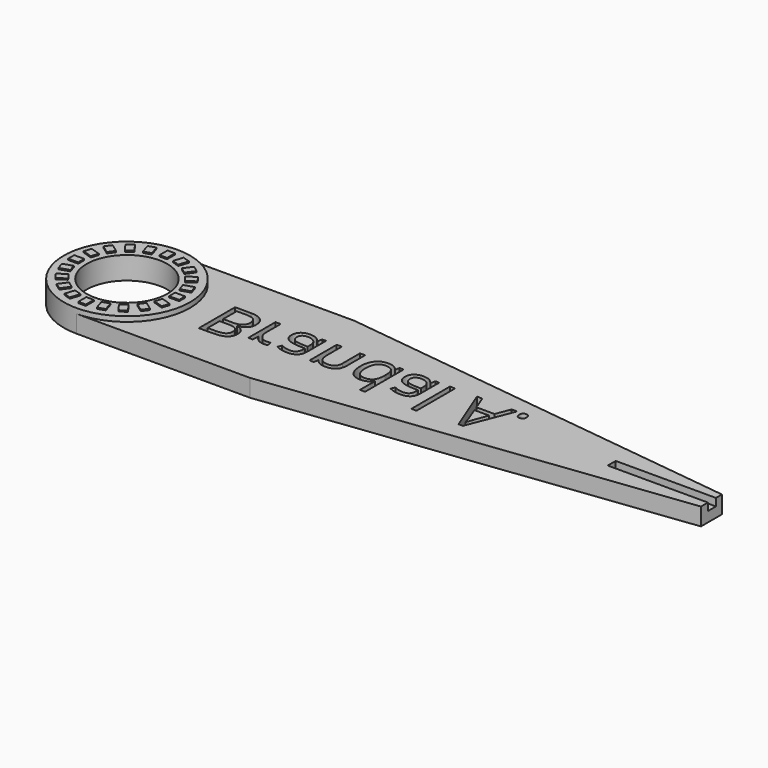
from build123d import *

# Parameters (mm, degrees)
F0_R         = 8.0699934722
F1_DEPTH     = 3.5
F2_R         = 12.6093648002
F2_R_2       = 8.0699934722
F3_DEPTH     = 1
F4_W         = 1.5
F4_H         = 2
F4_W_2       = 2
F4_H_2       = 1.5
F5_DEPTH     = 0.25
F6_W         = 20
F6_H         = 2
F7_DEPTH     = 1.5
F9_TEXT_SIZE = 12.6782884311
F10_DEPTH    = 4.751


# Not quite as in the source:
# - Text() gives the source's letters only with a copy of the font that has no kerning and outlines rounded to 1/6400 em; it was checked with that copy


with BuildPart() as f1:
    # F0 (on Top) → F1 (new body)
    with BuildSketch(Plane.XY):
        with BuildLine():
            Line((35.3062214407, 12.6093648002), (0, 12.6093648002))
            ThreePointArc((0, 12.6093648002), (-12.6093648002, 0), (0, -12.6093648002))
            Line((0, -12.6093648002), (34.6995617834, -12.6093648002))
            Line((34.6995617834, -12.6093648002), (116.6950058753, -2.616078641))
            Line((116.6950058753, -2.616078641), (116.6950058753, 2.616078641))
            Line((116.6950058753, 2.616078641), (35.3062214407, 12.6093648002))
        make_face()
        Circle(F0_R, mode=Mode.SUBTRACT)
    extrude(amount=F1_DEPTH)

    # F2 (on face) → F3 (join)
    with BuildSketch(Plane.XY.offset(3.5)):
        Circle(F2_R)
        Circle(F2_R_2, mode=Mode.SUBTRACT)
    extrude(amount=F3_DEPTH)

    # F4 (on face) → F5 (join)
    with BuildSketch(Plane.XY.offset(4.5)):
        with Locations((0, 10.0699934722)):
            Rectangle(F4_W, F4_H)
        Polygon((-2.7183706851, 10.7678329519), (-4.1449554595, 10.3043074603), (-3.5269214708, 8.4021944277), (-2.1003366963, 8.8657199193), align=None)
        Polygon((-5.9236144903, 9.4086757356), (-7.1371399818, 8.5269978571), (-5.9615694773, 6.9089638684), (-4.7480439857, 7.7906417468), align=None)
        Polygon((-8.5519798197, 7.1255656015), (-9.4336576981, 5.9120401099), (-7.8156237093, 4.7364696053), (-6.9339458309, 5.9499950969), align=None)
        Polygon((-10.3461839619, 4.1419892768), (-10.8097094535, 2.7154045023), (-8.9075964209, 2.0973705136), (-8.4440709293, 3.523955288), align=None)
        with Locations((-10.1305977146, 0)):
            Rectangle(F4_W_2, F4_H_2)
        Polygon((-10.8284371943, -2.7183706851), (-10.3649117027, -4.1449554595), (-8.4627986701, -3.5269214708), (-8.9263241617, -2.1003366963), align=None)
        Polygon((-9.469279978, -5.9236144903), (-8.5876020996, -7.1371399818), (-6.9695681108, -5.9615694773), (-7.8512459893, -4.7480439857), align=None)
        Polygon((-7.1861698439, -8.5519798197), (-5.9726443523, -9.4336576981), (-4.7970738477, -7.8156237093), (-6.0105993393, -6.9339458309), align=None)
        Polygon((-4.2025935192, -10.3461839619), (-2.7760087448, -10.8097094535), (-2.157974756, -8.9075964209), (-3.5845595305, -8.4440709293), align=None)
        with Locations((-0.0606042424, -10.1305977146)):
            Rectangle(F4_W, F4_H)
        Polygon((2.6577664427, -10.8284371943), (4.0843512171, -10.3649117027), (3.4663172284, -8.4627986701), (2.0397324539, -8.9263241617), align=None)
        Polygon((5.8630102478, -9.469279978), (7.0765357394, -8.5876020996), (5.9009652348, -6.9695681108), (4.6874397433, -7.8512459893), align=None)
        Polygon((8.4913755772, -7.1861698439), (9.3730534557, -5.9726443523), (7.7550194669, -4.7970738477), (6.8733415885, -6.0105993393), align=None)
        Polygon((10.2855797195, -4.2025935192), (10.749105211, -2.7760087448), (8.8469921784, -2.157974756), (8.3834666869, -3.5845595305), align=None)
        with Locations((10.0699934722, -0.0606042424)):
            Rectangle(F4_W_2, F4_H_2)
        Polygon((10.7678329519, 2.6577664427), (10.3043074603, 4.0843512171), (8.4021944277, 3.4663172284), (8.8657199193, 2.0397324539), align=None)
        Polygon((9.4086757356, 5.8630102478), (8.5269978571, 7.0765357394), (6.9089638684, 5.9009652348), (7.7906417468, 4.6874397433), align=None)
        Polygon((7.1255656015, 8.4913755772), (5.9120401099, 9.3730534557), (4.7364696053, 7.7550194669), (5.9499950969, 6.8733415885), align=None)
        Polygon((4.1419892768, 10.2855797195), (2.7154045023, 10.749105211), (2.0973705136, 8.8469921784), (3.523955288, 8.3834666869), align=None)
    extrude(amount=F5_DEPTH)

    # F6 (on face) → F7 (cut)
    with BuildSketch(Plane.XY.offset(3.5)):
        with Locations((106.6950058753, 0.116078641)):
            Rectangle(F6_W, F6_H)
    extrude(amount=-F7_DEPTH, mode=Mode.SUBTRACT)

    # F9 (on face) → F10 (cut, through all)
    with BuildSketch(Plane(origin=(0, 0, 0), x_dir=(1, 0, 0), z_dir=(0, 0, -1))):
        with Locations((16.6950058753, -4.5641838352)):
            Text('Brandal A.', F9_TEXT_SIZE, font='Open Sans', text_align=(TextAlign.LEFT, TextAlign.BOTTOM))
    extrude(amount=-F10_DEPTH, mode=Mode.SUBTRACT)


solid = f1.part
